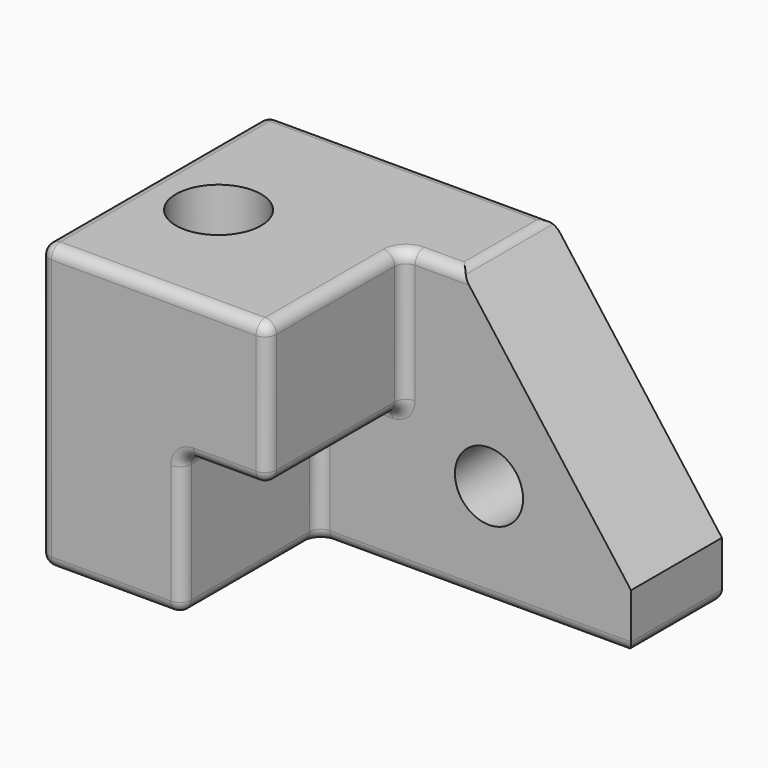
from build123d import *

# Parameters (mm, degrees)
F0_W        = 203.2
F0_H        = 127
F1_DEPTH    = 127
F3_DEPTH    = 25.4
F4_DEPTH    = 101.6
F5_T1_DEPTH = 575.1977482789
F6_R        = 5.08
F7_R        = 15.24
F8_DEPTH    = 50.8
F9_R        = 19.05
F10_DEPTH   = 127


# Not quite as in the source:
# - a fillet or chamfer that OpenCascade refuses, or shapes differently, is made with other operations: its cross-section is extruded or revolved along the edge and cut away or added


with BuildPart() as f1:
    # F0 (on Front) → F1 (new body)
    with BuildSketch(Plane.XZ):
        Rectangle(F0_W, F0_H)
    extrude(amount=F1_DEPTH)

    # F2 (on face) → F3 (join)
    with BuildSketch(Plane.XZ.offset(127)):
        Polygon((101.6, 63.5), (0, 63.5), (0, 0), (-38.1, 0), (-38.1, -63.5), (101.6, -63.5), align=None)
    extrude(amount=F3_DEPTH)

    # F4 (cut): a face of the model
    f4_faces = [f1.faces().sort_by_distance(p)[0] for p in [
        (39.7710526316, -152.4, -5.0131578947),
    ]]
    extrude(f4_faces, amount=-F4_DEPTH, mode=Mode.SUBTRACT)

    # F5: chamfer of 76.2 x 101.6 on 1 edges, made by hand

    # F5_s2 → F5_t1 (cut)
    with BuildSketch(Plane.XZ.offset(-262.1988741395)):
        Polygon((101.6, -38.1), (25.4, 63.5), (101.6, 63.5), align=None)
    extrude(amount=F5_T1_DEPTH, mode=Mode.SUBTRACT)

    # F6
    f6_edges = [f1.edges().sort_by_distance(p)[0] for p in [
        (-50.8, -127, 63.5),
        (0, -88.9, 63.5),
        (0, -127, 31.75),
        (-19.05, -127, 0),
        (-69.85, -127, -63.5),
        (-101.6, -127, 0),
        (-38.1, -127, -31.75),
        (-38.1, -88.9, -63.5),
        (31.75, -50.8, -63.5),
        (-38.1, -50.8, -31.75),
        (101.6, -25.4, -63.5),
        (0, 0, -63.5),
        (-101.6, 0, 0),
        (-101.6, -63.5, -63.5),
        (12.7, -50.8, 63.5),
        (25.4, -25.4, 63.5),
        (-38.1, 0, 63.5),
        (0, -88.9, 0),
        (-19.05, -50.8, 0),
        (-38.1, -88.9, 0),
        (-101.6, -63.5, 63.5),
        (0, -50.8, 31.75),
    ]]
    fillet(f6_edges, radius=F6_R)

    # F7 (on face) → F8 (cut, through all)
    with BuildSketch(Plane.XZ.offset(50.8)):
        with Locations((38.1, -17.78)):
            Circle(F7_R)
    extrude(amount=-F8_DEPTH, mode=Mode.SUBTRACT)

    # F9 (on face) → F10 (cut, through all)
    with BuildSketch(Plane.XY.offset(63.5)):
        with Locations((-68.58, -68.58)):
            Circle(F9_R)
    extrude(amount=-F10_DEPTH, mode=Mode.SUBTRACT)


solid = f1.part
